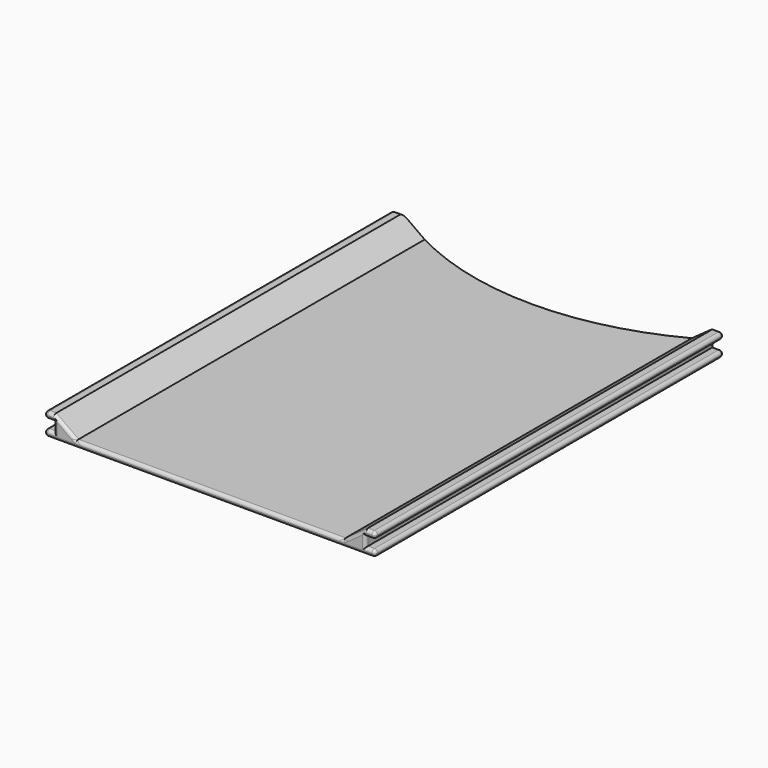
from build123d import *

# Parameters (mm, degrees)
F1_DEPTH       = 2
F2_W           = 10
F2_H           = 137
F3_DEPTH       = 5
F4_W           = 137
F4_H           = 3
F5_DEPTH       = 3
F6_W           = 137
F6_H           = 3
F7_DEPTH       = 3
F8_T4_DEPTH    = 173.1483869651
F8_T9_DEPTH    = 173.1483869651
F10_T1_DEPTH   = 134.9980686292
F10_T3_DEPTH   = 101.9980686292
F10_T5_DEPTH   = 1.9990343146
F10_T7_DEPTH   = 3
F10_T9_DEPTH   = 4.5014487279
F10_T11_DEPTH  = 4.5014487279
F10_T13_DEPTH  = 1.9990343146
F10_T15_DEPTH  = 11.5014487279
F10_T17_DEPTH  = 11.5014487279
F10_S21_W      = 1.1015022539
F10_S21_H      = 1.1015022539
F10_T22_DEPTH  = 1.101502254
F10_S27_W      = 1.1015022539
F10_S27_H      = 1.1015022539
F10_T28_DEPTH  = 1.101502254
F10_S33_W      = 1.1015022539
F10_S33_H      = 1.1015022539
F10_T34_DEPTH  = 1.101502254
F10_S39_W      = 1.1015022539
F10_S39_H      = 1.1015022539
F10_T40_DEPTH  = 1.101502254
F10_S45_W      = 1.1015022539
F10_S45_H      = 1.1015022539
F10_T46_DEPTH  = 1.101502254
F10_S51_W      = 1.1015022539
F10_S51_H      = 1.1015022539
F10_T52_DEPTH  = 1.101502254
F10_S57_W      = 1.1015022539
F10_S57_H      = 1.1015022539
F10_T58_DEPTH  = 1.101502254
F10_S63_W      = 1.1015022539
F10_S63_H      = 1.1015022539
F10_T64_DEPTH  = 1.101502254
F10_S69_W      = 1.1015022539
F10_S69_H      = 1.1015022539
F10_T70_DEPTH  = 1.101502254
F10_S75_W      = 1.1015022539
F10_S75_H      = 1.1015022539
F10_T76_DEPTH  = 1.101502254
F10_S81_W      = 1.1015022539
F10_S81_H      = 1.1015022539
F10_T82_DEPTH  = 1.101502254
F10_S87_W      = 1.1015022539
F10_S87_H      = 1.1015022539
F10_T88_DEPTH  = 1.101502254
F10_S93_W      = 1.1015022539
F10_S93_H      = 1.1015022539
F10_T94_DEPTH  = 1.101502254
F10_S99_W      = 1.1015022539
F10_S99_H      = 1.1015022539
F10_T100_DEPTH = 1.101502254
F10_S105_W     = 1.1015022539
F10_S105_H     = 1.1015022539
F10_T106_DEPTH = 1.101502254
F10_S111_W     = 1.1015022539
F10_S111_H     = 1.1015022539
F10_T112_DEPTH = 1.101502254
F10_T118_DEPTH = 13.6071540938
F10_T123_DEPTH = 89.0048288267
F10_T129_DEPTH = 13.6071540938
F10_T132_ANGLE = 58.8229405879
F10_T137_DEPTH = 4.5014487279
F10_T141_DEPTH = 5.5024144134
F10_T149_DEPTH = 5.5024144134
F10_T155_DEPTH = 4.5014487279
F10_T163_DEPTH = 13.6071540938
F10_T168_DEPTH = 89.0048288267
F10_T175_DEPTH = 13.6071540938
F10_T180_DEPTH = 89.0048288267
F10_T187_DEPTH = 5.5024144134
F10_T193_DEPTH = 4.5014487279
F10_T201_DEPTH = 4.5014487279
F10_T205_DEPTH = 5.5024144134
F10_T213_DEPTH = 4.5014487279
F10_T218_DEPTH = 5.5024144134
F10_T227_DEPTH = 5.5024144134
F10_T232_DEPTH = 4.5014487279
F10_T239_DEPTH = 4.5014487279
F10_T243_DEPTH = 5.5024144134
F10_T251_DEPTH = 5.5024144134
F10_T257_DEPTH = 4.5014487279


# Not quite as in the source:
# - a fillet or chamfer that OpenCascade refuses, or shapes differently, is made with other operations: its cross-section is extruded or revolved along the edge and cut away or added
# - two fillets or chamfers of one size are made in one step


with BuildPart() as f1:
    # F0 (on Top) → F1 (new body)
    with BuildSketch(Plane.XY):
        with BuildLine():
            Line((-52, -68.5), (0, -68.5))
            Line((0, -68.5), (52, -68.5))
            Line((52, -68.5), (52, 68.5))
            Line((52, 68.5), (42, 68.5))
            ThreePointArc((42, 68.5), (0, 58.0989949685), (-42, 68.5))
            Line((-42, 68.5), (-52, 68.5))
            Line((-52, 68.5), (-52, -68.5))
        make_face()
    extrude(amount=F1_DEPTH)

    # F2 (on face) → F3 (join)
    with BuildSketch(Plane.XY.offset(2)):
        with Locations((-47, 0)):
            Rectangle(F2_W, F2_H)
        with Locations((47, 0)):
            Rectangle(F2_W, F2_H)
    extrude(amount=F3_DEPTH)

    # F4 (on face) → F5 (cut)
    with BuildSketch(Plane(origin=(-52, 0, 0), x_dir=(0, -1, 0), z_dir=(-1, 0, 0))):
        with Locations((0, 3.5)):
            Rectangle(F4_W, F4_H)
    extrude(amount=-F5_DEPTH, mode=Mode.SUBTRACT)

    # F6 (on face) → F7 (cut)
    with BuildSketch(Plane.YZ.offset(52)):
        with Locations((0, 3.5)):
            Rectangle(F6_W, F6_H)
    extrude(amount=-F7_DEPTH, mode=Mode.SUBTRACT)

    # F8: chamfer of 7 x 5 on 2 edges, made by hand


with BuildPart() as f8_tool2:
    # F8_s3 → F8_t4 (new body)
    with BuildSketch(Plane.XZ.offset(86.5741934825)):
        Polygon((-49, 7), (-42, 2), (-42, 7), align=None)
    extrude(amount=-F8_T4_DEPTH)

    split(bisect_by=Plane.XY.offset(2), keep=Keep.TOP)


with BuildPart() as f1_1:
    add(f1.part)

    # F8_t1: cut F8_tool2
    add(f8_tool2.part, mode=Mode.SUBTRACT)


with BuildPart() as f8_tool7:
    # F8_s8 → F8_t9 (new body)
    with BuildSketch(Plane.XZ.offset(-86.5741934825)):
        Polygon((49, 7), (42, 2), (42, 7), align=None)
    extrude(amount=F8_T9_DEPTH)

    split(bisect_by=Plane.XY.offset(2), keep=Keep.TOP)


with BuildPart() as f1_2:
    add(f1_1.part)

    # F8_t6: cut F8_tool7
    add(f8_tool7.part, mode=Mode.SUBTRACT)

    # F10: fillet of radius 1 on 39 edges, made by hand

    # F10_s2 → F10_t1 (cut)
    with BuildSketch(Plane.XZ.offset(-67.4990343146)):
        with BuildLine():
            ThreePointArc((52.0004, 0.9990343146), (51.7071067812, 1.7071067812), (50.9990343146, 2.0004))
            Line((50.9990343146, 2.0004), (50.9990343146, 2.1005365685))
            ThreePointArc((50.9990343146, 2.1005365685), (51.4995171573, 2.1001365685), (52, 2.1001365685))
            Line((52, 2.1001365685), (52.1001365685, 2))
            ThreePointArc((52.1001365685, 2), (52.1001365685, 1.4995171573), (52.1005365685, 0.9990343146))
            Line((52.1005365685, 0.9990343146), (52.0004, 0.9990343146))
        make_face()
        with BuildLine():
            ThreePointArc((50.9990343146, -0.0004), (51.7071067812, 0.2928932188), (52.0004, 1.0009656854))
            Line((52.0004, 1.0009656854), (52.1005365685, 1.0009656854))
            ThreePointArc((52.1005365685, 1.0009656854), (52.1001365685, 0.5004828427), (52.1001365685, 0))
            Line((52.1001365685, 0), (52, -0.1001365685))
            ThreePointArc((52, -0.1001365685), (51.4995171573, -0.1001365685), (50.9990343146, -0.1005365685))
            Line((50.9990343146, -0.1005365685), (50.9990343146, -0.0004))
        make_face()
        with BuildLine():
            ThreePointArc((52.0004, 5.9990343146), (51.7071067812, 6.7071067812), (50.9990343146, 7.0004))
            Line((50.9990343146, 7.0004), (50.9990343146, 7.1005365685))
            ThreePointArc((50.9990343146, 7.1005365685), (51.4995171573, 7.1001365685), (52, 7.1001365685))
            Line((52, 7.1001365685), (52.1001365685, 7))
            ThreePointArc((52.1001365685, 7), (52.1001365685, 6.4995171573), (52.1005365685, 5.9990343146))
            Line((52.1005365685, 5.9990343146), (52.0004, 5.9990343146))
        make_face()
        with BuildLine():
            ThreePointArc((50.9990343146, 4.9996), (51.7071067812, 5.2928932188), (52.0004, 6.0009656854))
            Line((52.0004, 6.0009656854), (52.1005365685, 6.0009656854))
            ThreePointArc((52.1005365685, 6.0009656854), (52.1001365685, 5.5004828427), (52.1001365685, 5))
            Line((52.1001365685, 5), (52, 4.8998634315))
            ThreePointArc((52, 4.8998634315), (51.4995171573, 4.8998634315), (50.9990343146, 4.8994634315))
            Line((50.9990343146, 4.8994634315), (50.9990343146, 4.9996))
        make_face()
        with BuildLine():
            ThreePointArc((-52.0004, 5.9990343146), (-51.7071067812, 6.7071067812), (-50.9990343146, 7.0004))
            Line((-50.9990343146, 7.0004), (-50.9990343146, 7.1005365685))
            ThreePointArc((-50.9990343146, 7.1005365685), (-51.4995171573, 7.1001365685), (-52, 7.1001365685))
            Line((-52, 7.1001365685), (-52.1001365685, 7))
            ThreePointArc((-52.1001365685, 7), (-52.1001365685, 6.4995171573), (-52.1005365685, 5.9990343146))
            Line((-52.1005365685, 5.9990343146), (-52.0004, 5.9990343146))
        make_face()
        with BuildLine():
            ThreePointArc((-50.9990343146, 4.9996), (-51.7071067812, 5.2928932188), (-52.0004, 6.0009656854))
            Line((-52.0004, 6.0009656854), (-52.1005365685, 6.0009656854))
            ThreePointArc((-52.1005365685, 6.0009656854), (-52.1001365685, 5.5004828427), (-52.1001365685, 5))
            Line((-52.1001365685, 5), (-52, 4.8998634315))
            ThreePointArc((-52, 4.8998634315), (-51.4995171573, 4.8998634315), (-50.9990343146, 4.8994634315))
            Line((-50.9990343146, 4.8994634315), (-50.9990343146, 4.9996))
        make_face()
        with BuildLine():
            ThreePointArc((-52.0004, 0.9990343146), (-51.7071067812, 1.7071067812), (-50.9990343146, 2.0004))
            Line((-50.9990343146, 2.0004), (-50.9990343146, 2.1005365685))
            ThreePointArc((-50.9990343146, 2.1005365685), (-51.4995171573, 2.1001365685), (-52, 2.1001365685))
            Line((-52, 2.1001365685), (-52.1001365685, 2))
            ThreePointArc((-52.1001365685, 2), (-52.1001365685, 1.4995171573), (-52.1005365685, 0.9990343146))
            Line((-52.1005365685, 0.9990343146), (-52.0004, 0.9990343146))
        make_face()
        with BuildLine():
            ThreePointArc((-50.9990343146, -0.0004), (-51.7071067812, 0.2928932188), (-52.0004, 1.0009656854))
            Line((-52.0004, 1.0009656854), (-52.1005365685, 1.0009656854))
            ThreePointArc((-52.1005365685, 1.0009656854), (-52.1001365685, 0.5004828427), (-52.1001365685, 0))
            Line((-52.1001365685, 0), (-52, -0.1001365685))
            ThreePointArc((-52, -0.1001365685), (-51.4995171573, -0.1001365685), (-50.9990343146, -0.1005365685))
            Line((-50.9990343146, -0.1005365685), (-50.9990343146, -0.0004))
        make_face()
    extrude(amount=F10_T1_DEPTH, mode=Mode.SUBTRACT)

    # F10_s4 → F10_t3 (cut)
    with BuildSketch(Plane.YZ.offset(-50.9990343146)):
        with BuildLine():
            ThreePointArc((-67.4990343146, -0.0004), (-68.2071067812, 0.2928932188), (-68.5004, 1.0009656854))
            Line((-68.5004, 1.0009656854), (-68.6005365685, 1.0009656854))
            ThreePointArc((-68.6005365685, 1.0009656854), (-68.6001365685, 0.5004828427), (-68.6001365685, 0))
            Line((-68.6001365685, 0), (-68.5, -0.1001365685))
            ThreePointArc((-68.5, -0.1001365685), (-67.9995171573, -0.1001365685), (-67.4990343146, -0.1005365685))
            Line((-67.4990343146, -0.1005365685), (-67.4990343146, -0.0004))
        make_face()
    extrude(amount=F10_T3_DEPTH, mode=Mode.SUBTRACT)

    # F10_s6 → F10_t5 (cut)
    with BuildSketch(Plane.YZ.offset(49)):
        with BuildLine():
            ThreePointArc((-68.5004, 0.9990343146), (-68.2071067812, 1.7071067812), (-67.4990343146, 2.0004))
            Line((-67.4990343146, 2.0004), (-67.4990343146, 2.1005365685))
            ThreePointArc((-67.4990343146, 2.1005365685), (-67.9995171573, 2.1001365685), (-68.5, 2.1001365685))
            Line((-68.5, 2.1001365685), (-68.6001365685, 2))
            ThreePointArc((-68.6001365685, 2), (-68.6001365685, 1.4995171573), (-68.6005365685, 0.9990343146))
            Line((-68.6005365685, 0.9990343146), (-68.5004, 0.9990343146))
        make_face()
        with BuildLine():
            ThreePointArc((-68.5004, 6.0009656854), (-68.2071067812, 5.2928932188), (-67.4990343146, 4.9996))
            Line((-67.4990343146, 4.9996), (-67.4990343146, 4.8994634315))
            ThreePointArc((-67.4990343146, 4.8994634315), (-67.9995171573, 4.8998634315), (-68.5, 4.8998634315))
            Line((-68.5, 4.8998634315), (-68.6001365685, 5))
            ThreePointArc((-68.6001365685, 5), (-68.6001365685, 5.5004828427), (-68.6005365685, 6.0009656854))
            Line((-68.6005365685, 6.0009656854), (-68.5004, 6.0009656854))
        make_face()
        with BuildLine():
            ThreePointArc((68.5004, 6.0009656854), (68.2071067812, 5.2928932188), (67.4990343146, 4.9996))
            Line((67.4990343146, 4.9996), (67.4990343146, 4.8994634315))
            ThreePointArc((67.4990343146, 4.8994634315), (67.9995171573, 4.8998634315), (68.5, 4.8998634315))
            Line((68.5, 4.8998634315), (68.6001365685, 5))
            ThreePointArc((68.6001365685, 5), (68.6001365685, 5.5004828427), (68.6005365685, 6.0009656854))
            Line((68.6005365685, 6.0009656854), (68.5004, 6.0009656854))
        make_face()
        with BuildLine():
            ThreePointArc((68.5004, 0.9990343146), (68.2071067812, 1.7071067812), (67.4990343146, 2.0004))
            Line((67.4990343146, 2.0004), (67.4990343146, 2.1005365685))
            ThreePointArc((67.4990343146, 2.1005365685), (67.9995171573, 2.1001365685), (68.5, 2.1001365685))
            Line((68.5, 2.1001365685), (68.6001365685, 2))
            ThreePointArc((68.6001365685, 2), (68.6001365685, 1.4995171573), (68.6005365685, 0.9990343146))
            Line((68.6005365685, 0.9990343146), (68.5004, 0.9990343146))
        make_face()
    extrude(amount=F10_T5_DEPTH, mode=Mode.SUBTRACT)

    # F10_s8 → F10_t7 (cut)
    with BuildSketch(Plane.XY.offset(2)):
        with BuildLine():
            ThreePointArc((47.9990343146, -68.5004), (48.7071067812, -68.2071067812), (49.0004, -67.4990343146))
            Line((49.0004, -67.4990343146), (49.1005365685, -67.4990343146))
            ThreePointArc((49.1005365685, -67.4990343146), (49.1001365685, -67.9995171573), (49.1001365685, -68.5))
            Line((49.1001365685, -68.5), (49, -68.6001365685))
            ThreePointArc((49, -68.6001365685), (48.4995171573, -68.6001365685), (47.9990343146, -68.6005365685))
            Line((47.9990343146, -68.6005365685), (47.9990343146, -68.5004))
        make_face()
        with BuildLine():
            ThreePointArc((-49.0004, -67.4990343146), (-48.7071067812, -68.2071067812), (-47.9990343146, -68.5004))
            Line((-47.9990343146, -68.5004), (-47.9990343146, -68.6005365685))
            ThreePointArc((-47.9990343146, -68.6005365685), (-48.4995171573, -68.6001365685), (-49, -68.6001365685))
            Line((-49, -68.6001365685), (-49.1001365685, -68.5))
            ThreePointArc((-49.1001365685, -68.5), (-49.1001365685, -67.9995171573), (-49.1005365685, -67.4990343146))
            Line((-49.1005365685, -67.4990343146), (-49.0004, -67.4990343146))
        make_face()
        with BuildLine():
            ThreePointArc((47.9990343146, 68.5004), (48.7071067812, 68.2071067812), (49.0004, 67.4990343146))
            Line((49.0004, 67.4990343146), (49.1005365685, 67.4990343146))
            ThreePointArc((49.1005365685, 67.4990343146), (49.1001365685, 67.9995171573), (49.1001365685, 68.5))
            Line((49.1001365685, 68.5), (49, 68.6001365685))
            ThreePointArc((49, 68.6001365685), (48.4995171573, 68.6001365685), (47.9990343146, 68.6005365685))
            Line((47.9990343146, 68.6005365685), (47.9990343146, 68.5004))
        make_face()
        with BuildLine():
            ThreePointArc((-47.9990343146, 68.5004), (-48.7071067812, 68.2071067812), (-49.0004, 67.4990343146))
            Line((-49.0004, 67.4990343146), (-49.1005365685, 67.4990343146))
            ThreePointArc((-49.1005365685, 67.4990343146), (-49.1001365685, 67.9995171573), (-49.1001365685, 68.5))
            Line((-49.1001365685, 68.5), (-49, 68.6001365685))
            ThreePointArc((-49, 68.6001365685), (-48.4995171573, 68.6001365685), (-47.9990343146, 68.6005365685))
            Line((-47.9990343146, 68.6005365685), (-47.9990343146, 68.5004))
        make_face()
    extrude(amount=F10_T7_DEPTH, mode=Mode.SUBTRACT)

    # F10_s10 → F10_t9 (cut)
    with BuildSketch(Plane.YZ.offset(46.4975855866)):
        with BuildLine():
            ThreePointArc((-68.5004, 5.9990343146), (-68.2071067812, 6.7071067812), (-67.4990343146, 7.0004))
            Line((-67.4990343146, 7.0004), (-67.4990343146, 7.1005365685))
            ThreePointArc((-67.4990343146, 7.1005365685), (-67.9995171573, 7.1001365685), (-68.5, 7.1001365685))
            Line((-68.5, 7.1001365685), (-68.6001365685, 7))
            ThreePointArc((-68.6001365685, 7), (-68.6001365685, 6.4995171573), (-68.6005365685, 5.9990343146))
            Line((-68.6005365685, 5.9990343146), (-68.5004, 5.9990343146))
        make_face()
        with BuildLine():
            ThreePointArc((68.5004, 5.9990343146), (68.2071067812, 6.7071067812), (67.4990343146, 7.0004))
            Line((67.4990343146, 7.0004), (67.4990343146, 7.1005365685))
            ThreePointArc((67.4990343146, 7.1005365685), (67.9995171573, 7.1001365685), (68.5, 7.1001365685))
            Line((68.5, 7.1001365685), (68.6001365685, 7))
            ThreePointArc((68.6001365685, 7), (68.6001365685, 6.4995171573), (68.6005365685, 5.9990343146))
            Line((68.6005365685, 5.9990343146), (68.5004, 5.9990343146))
        make_face()
    extrude(amount=F10_T9_DEPTH, mode=Mode.SUBTRACT)

    # F10_s12 → F10_t11 (cut)
    with BuildSketch(Plane.YZ.offset(-50.9990343146)):
        with BuildLine():
            ThreePointArc((-67.4990343146, 7.0004), (-68.2071067812, 6.7071067812), (-68.5004, 5.9990343146))
            Line((-68.5004, 5.9990343146), (-68.6005365685, 5.9990343146))
            ThreePointArc((-68.6005365685, 5.9990343146), (-68.6001365685, 6.4995171573), (-68.6001365685, 7))
            Line((-68.6001365685, 7), (-68.5, 7.1001365685))
            ThreePointArc((-68.5, 7.1001365685), (-67.9995171573, 7.1001365685), (-67.4990343146, 7.1005365685))
            Line((-67.4990343146, 7.1005365685), (-67.4990343146, 7.0004))
        make_face()
        with BuildLine():
            ThreePointArc((68.5004, 5.9990343146), (68.2071067812, 6.7071067812), (67.4990343146, 7.0004))
            Line((67.4990343146, 7.0004), (67.4990343146, 7.1005365685))
            ThreePointArc((67.4990343146, 7.1005365685), (67.9995171573, 7.1001365685), (68.5, 7.1001365685))
            Line((68.5, 7.1001365685), (68.6001365685, 7))
            ThreePointArc((68.6001365685, 7), (68.6001365685, 6.4995171573), (68.6005365685, 5.9990343146))
            Line((68.6005365685, 5.9990343146), (68.5004, 5.9990343146))
        make_face()
    extrude(amount=F10_T11_DEPTH, mode=Mode.SUBTRACT)

    # F10_s14 → F10_t13 (cut)
    with BuildSketch(Plane.YZ.offset(-50.9990343146)):
        with BuildLine():
            ThreePointArc((-67.4990343146, 4.9996), (-68.2071067812, 5.2928932188), (-68.5004, 6.0009656854))
            Line((-68.5004, 6.0009656854), (-68.6005365685, 6.0009656854))
            ThreePointArc((-68.6005365685, 6.0009656854), (-68.6001365685, 5.5004828427), (-68.6001365685, 5))
            Line((-68.6001365685, 5), (-68.5, 4.8998634315))
            ThreePointArc((-68.5, 4.8998634315), (-67.9995171573, 4.8998634315), (-67.4990343146, 4.8994634315))
            Line((-67.4990343146, 4.8994634315), (-67.4990343146, 4.9996))
        make_face()
        with BuildLine():
            ThreePointArc((-67.4990343146, 2.0004), (-68.2071067812, 1.7071067812), (-68.5004, 0.9990343146))
            Line((-68.5004, 0.9990343146), (-68.6005365685, 0.9990343146))
            ThreePointArc((-68.6005365685, 0.9990343146), (-68.6001365685, 1.4995171573), (-68.6001365685, 2))
            Line((-68.6001365685, 2), (-68.5, 2.1001365685))
            ThreePointArc((-68.5, 2.1001365685), (-67.9995171573, 2.1001365685), (-67.4990343146, 2.1005365685))
            Line((-67.4990343146, 2.1005365685), (-67.4990343146, 2.0004))
        make_face()
        with BuildLine():
            ThreePointArc((68.5004, 0.9990343146), (68.2071067812, 1.7071067812), (67.4990343146, 2.0004))
            Line((67.4990343146, 2.0004), (67.4990343146, 2.1005365685))
            ThreePointArc((67.4990343146, 2.1005365685), (67.9995171573, 2.1001365685), (68.5, 2.1001365685))
            Line((68.5, 2.1001365685), (68.6001365685, 2))
            ThreePointArc((68.6001365685, 2), (68.6001365685, 1.4995171573), (68.6005365685, 0.9990343146))
            Line((68.6005365685, 0.9990343146), (68.5004, 0.9990343146))
        make_face()
        with BuildLine():
            ThreePointArc((68.5004, 6.0009656854), (68.2071067812, 5.2928932188), (67.4990343146, 4.9996))
            Line((67.4990343146, 4.9996), (67.4990343146, 4.8994634315))
            ThreePointArc((67.4990343146, 4.8994634315), (67.9995171573, 4.8998634315), (68.5, 4.8998634315))
            Line((68.5, 4.8998634315), (68.6001365685, 5))
            ThreePointArc((68.6001365685, 5), (68.6001365685, 5.5004828427), (68.6005365685, 6.0009656854))
            Line((68.6005365685, 6.0009656854), (68.5004, 6.0009656854))
        make_face()
    extrude(amount=F10_T13_DEPTH, mode=Mode.SUBTRACT)

    # F10_s16 → F10_t15 (cut)
    with BuildSketch(Plane.YZ.offset(39.4975855866)):
        with BuildLine():
            ThreePointArc((67.4990343146, -0.0004), (68.2071067812, 0.2928932188), (68.5004, 1.0009656854))
            Line((68.5004, 1.0009656854), (68.6005365685, 1.0009656854))
            ThreePointArc((68.6005365685, 1.0009656854), (68.6001365685, 0.5004828427), (68.6001365685, 0))
            Line((68.6001365685, 0), (68.5, -0.1001365685))
            ThreePointArc((68.5, -0.1001365685), (67.9995171573, -0.1001365685), (67.4990343146, -0.1005365685))
            Line((67.4990343146, -0.1005365685), (67.4990343146, -0.0004))
        make_face()
    extrude(amount=F10_T15_DEPTH, mode=Mode.SUBTRACT)

    # F10_s18 → F10_t17 (cut)
    with BuildSketch(Plane.YZ.offset(-50.9990343146)):
        with BuildLine():
            ThreePointArc((68.5004, 1.0009656854), (68.2071067812, 0.2928932188), (67.4990343146, -0.0004))
            Line((67.4990343146, -0.0004), (67.4990343146, -0.1005365685))
            ThreePointArc((67.4990343146, -0.1005365685), (67.9995171573, -0.1001365685), (68.5, -0.1001365685))
            Line((68.5, -0.1001365685), (68.6001365685, 0))
            ThreePointArc((68.6001365685, 0), (68.6001365685, 0.5004828427), (68.6005365685, 1.0009656854))
            Line((68.6005365685, 1.0009656854), (68.5004, 1.0009656854))
        make_face()
    extrude(amount=F10_T17_DEPTH, mode=Mode.SUBTRACT)


with BuildPart() as f10_tool20:
    # F10_s21 → F10_t22 (new body)
    with BuildSketch(Plane.XZ.offset(67.4990343146)):
        with Locations((51.5497854416, 1.5497854416)):
            Rectangle(F10_S21_W, F10_S21_H)
    extrude(amount=F10_T22_DEPTH)

    # F10_s23 → F10_t24 (revolve, cut)
    with BuildSketch(Plane(origin=(50.9990343146, -67.4990343146, 0.9990343146), x_dir=(-0.7071067812, 0, -0.7071067812), z_dir=(-0.7071067812, 0, 0.7071067812))):
        with BuildLine():
            ThreePointArc((0, -1.0013656854), (1.0013656854, 0), (0, 1.0013656854))
            Line((0, 1.0013656854), (0, -1.0013656854))
        make_face()
    revolve(axis=Axis((50.9990343146, -67.4990343146, 0.9990343146), (0, -1, 0)), mode=Mode.SUBTRACT)


with BuildPart() as f1_3:
    add(f1_2.part)

    # F10_t19: cut F10_tool20
    add(f10_tool20.part, mode=Mode.SUBTRACT)


with BuildPart() as f10_tool26:
    # F10_s27 → F10_t28 (new body)
    with BuildSketch(Plane.YZ.offset(50.9990343146)):
        with Locations((68.0497854416, 1.5497854416)):
            Rectangle(F10_S27_W, F10_S27_H)
    extrude(amount=F10_T28_DEPTH)

    # F10_s29 → F10_t30 (revolve, cut)
    with BuildSketch(Plane(origin=(50.9990343146, 67.4990343146, 0.9990343146), x_dir=(0, -0.7071067812, -0.7071067812), z_dir=(0, -0.7071067812, 0.7071067812))):
        with BuildLine():
            ThreePointArc((0, -1.0013656854), (1.0013656854, 0), (0, 1.0013656854))
            Line((0, 1.0013656854), (0, -1.0013656854))
        make_face()
    revolve(axis=Axis((50.9990343146, 67.4990343146, 0.9990343146), (1, 0, 0)), mode=Mode.SUBTRACT)


with BuildPart() as f1_4:
    add(f1_3.part)

    # F10_t25: cut F10_tool26
    add(f10_tool26.part, mode=Mode.SUBTRACT)


with BuildPart() as f10_tool32:
    # F10_s33 → F10_t34 (new body)
    with BuildSketch(Plane.XY.offset(1.0009656854)):
        with Locations((51.5497854416, -68.0497854416)):
            Rectangle(F10_S33_W, F10_S33_H)
    extrude(amount=-F10_T34_DEPTH)

    # F10_s35 → F10_t36 (revolve, cut)
    with BuildSketch(Plane(origin=(50.9990343146, -67.4990343146, 1.0009656854), x_dir=(-0.7071067812, 0.7071067812, 0), z_dir=(-0.7071067812, -0.7071067812, 0))):
        with BuildLine():
            ThreePointArc((0, -1.0013656854), (1.0013656854, 0), (0, 1.0013656854))
            Line((0, 1.0013656854), (0, -1.0013656854))
        make_face()
    revolve(axis=Axis((50.9990343146, -67.4990343146, 1.0009656854), (0, 0, -1)), mode=Mode.SUBTRACT)


with BuildPart() as f1_5:
    add(f1_4.part)

    # F10_t31: cut F10_tool32
    add(f10_tool32.part, mode=Mode.SUBTRACT)


with BuildPart() as f10_tool38:
    # F10_s39 → F10_t40 (new body)
    with BuildSketch(Plane.XY.offset(1.0009656854)):
        with Locations((51.5497854416, 68.0497854416)):
            Rectangle(F10_S39_W, F10_S39_H)
    extrude(amount=-F10_T40_DEPTH)

    # F10_s41 → F10_t42 (revolve, cut)
    with BuildSketch(Plane(origin=(50.9990343146, 67.4990343146, 1.0009656854), x_dir=(-0.7071067812, -0.7071067812, 0), z_dir=(0.7071067812, -0.7071067812, 0))):
        with BuildLine():
            ThreePointArc((0, -1.0013656854), (1.0013656854, 0), (0, 1.0013656854))
            Line((0, 1.0013656854), (0, -1.0013656854))
        make_face()
    revolve(axis=Axis((50.9990343146, 67.4990343146, 1.0009656854), (0, 0, -1)), mode=Mode.SUBTRACT)


with BuildPart() as f1_6:
    add(f1_5.part)

    # F10_t37: cut F10_tool38
    add(f10_tool38.part, mode=Mode.SUBTRACT)


with BuildPart() as f10_tool44:
    # F10_s45 → F10_t46 (new body)
    with BuildSketch(Plane.YZ.offset(50.9990343146)):
        with Locations((-68.0497854416, 6.5497854416)):
            Rectangle(F10_S45_W, F10_S45_H)
    extrude(amount=F10_T46_DEPTH)

    # F10_s47 → F10_t48 (revolve, cut)
    with BuildSketch(Plane(origin=(50.9990343146, -67.4990343146, 5.9990343146), x_dir=(0, 0.7071067812, -0.7071067812), z_dir=(0, -0.7071067812, -0.7071067812))):
        with BuildLine():
            ThreePointArc((0, -1.0013656854), (1.0013656854, 0), (0, 1.0013656854))
            Line((0, 1.0013656854), (0, -1.0013656854))
        make_face()
    revolve(axis=Axis((50.9990343146, -67.4990343146, 5.9990343146), (1, 0, 0)), mode=Mode.SUBTRACT)


with BuildPart() as f1_7:
    add(f1_6.part)

    # F10_t43: cut F10_tool44
    add(f10_tool44.part, mode=Mode.SUBTRACT)


with BuildPart() as f10_tool50:
    # F10_s51 → F10_t52 (new body)
    with BuildSketch(Plane.YZ.offset(50.9990343146)):
        with Locations((68.0497854416, 6.5497854416)):
            Rectangle(F10_S51_W, F10_S51_H)
    extrude(amount=F10_T52_DEPTH)

    # F10_s53 → F10_t54 (revolve, cut)
    with BuildSketch(Plane(origin=(50.9990343146, 67.4990343146, 5.9990343146), x_dir=(0, -0.7071067812, -0.7071067812), z_dir=(0, -0.7071067812, 0.7071067812))):
        with BuildLine():
            ThreePointArc((0, -1.0013656854), (1.0013656854, 0), (0, 1.0013656854))
            Line((0, 1.0013656854), (0, -1.0013656854))
        make_face()
    revolve(axis=Axis((50.9990343146, 67.4990343146, 5.9990343146), (1, 0, 0)), mode=Mode.SUBTRACT)


with BuildPart() as f1_8:
    add(f1_7.part)

    # F10_t49: cut F10_tool50
    add(f10_tool50.part, mode=Mode.SUBTRACT)


with BuildPart() as f10_tool56:
    # F10_s57 → F10_t58 (new body)
    with BuildSketch(Plane.XY.offset(6.0009656854)):
        with Locations((51.5497854416, 68.0497854416)):
            Rectangle(F10_S57_W, F10_S57_H)
    extrude(amount=-F10_T58_DEPTH)

    # F10_s59 → F10_t60 (revolve, cut)
    with BuildSketch(Plane(origin=(50.9990343146, 67.4990343146, 6.0009656854), x_dir=(-0.7071067812, -0.7071067812, 0), z_dir=(0.7071067812, -0.7071067812, 0))):
        with BuildLine():
            ThreePointArc((0, -1.0013656854), (1.0013656854, 0), (0, 1.0013656854))
            Line((0, 1.0013656854), (0, -1.0013656854))
        make_face()
    revolve(axis=Axis((50.9990343146, 67.4990343146, 6.0009656854), (0, 0, -1)), mode=Mode.SUBTRACT)


with BuildPart() as f1_9:
    add(f1_8.part)

    # F10_t55: cut F10_tool56
    add(f10_tool56.part, mode=Mode.SUBTRACT)


with BuildPart() as f10_tool62:
    # F10_s63 → F10_t64 (new body)
    with BuildSketch(Plane.XY.offset(6.0009656854)):
        with Locations((51.5497854416, -68.0497854416)):
            Rectangle(F10_S63_W, F10_S63_H)
    extrude(amount=-F10_T64_DEPTH)

    # F10_s65 → F10_t66 (revolve, cut)
    with BuildSketch(Plane(origin=(50.9990343146, -67.4990343146, 6.0009656854), x_dir=(-0.7071067812, 0.7071067812, 0), z_dir=(-0.7071067812, -0.7071067812, 0))):
        with BuildLine():
            ThreePointArc((0, -1.0013656854), (1.0013656854, 0), (0, 1.0013656854))
            Line((0, 1.0013656854), (0, -1.0013656854))
        make_face()
    revolve(axis=Axis((50.9990343146, -67.4990343146, 6.0009656854), (0, 0, -1)), mode=Mode.SUBTRACT)


with BuildPart() as f1_10:
    add(f1_9.part)

    # F10_t61: cut F10_tool62
    add(f10_tool62.part, mode=Mode.SUBTRACT)


with BuildPart() as f10_tool68:
    # F10_s69 → F10_t70 (new body)
    with BuildSketch(Plane.XZ.offset(-67.4990343146)):
        with Locations((-51.5497854416, 6.5497854416)):
            Rectangle(F10_S69_W, F10_S69_H)
    extrude(amount=-F10_T70_DEPTH)

    # F10_s71 → F10_t72 (revolve, cut)
    with BuildSketch(Plane(origin=(-50.9990343146, 67.4990343146, 5.9990343146), x_dir=(0.7071067812, 0, -0.7071067812), z_dir=(0.7071067812, 0, 0.7071067812))):
        with BuildLine():
            ThreePointArc((0, -1.0013656854), (1.0013656854, 0), (0, 1.0013656854))
            Line((0, 1.0013656854), (0, -1.0013656854))
        make_face()
    revolve(axis=Axis((-50.9990343146, 67.4990343146, 5.9990343146), (0, 1, 0)), mode=Mode.SUBTRACT)


with BuildPart() as f1_11:
    add(f1_10.part)

    # F10_t67: cut F10_tool68
    add(f10_tool68.part, mode=Mode.SUBTRACT)


with BuildPart() as f10_tool74:
    # F10_s75 → F10_t76 (new body)
    with BuildSketch(Plane.XZ.offset(67.4990343146)):
        with Locations((-51.5497854416, 6.5497854416)):
            Rectangle(F10_S75_W, F10_S75_H)
    extrude(amount=F10_T76_DEPTH)

    # F10_s77 → F10_t78 (revolve, cut)
    with BuildSketch(Plane(origin=(-50.9990343146, -67.4990343146, 5.9990343146), x_dir=(0.7071067812, 0, -0.7071067812), z_dir=(-0.7071067812, 0, -0.7071067812))):
        with BuildLine():
            ThreePointArc((0, -1.0013656854), (1.0013656854, 0), (0, 1.0013656854))
            Line((0, 1.0013656854), (0, -1.0013656854))
        make_face()
    revolve(axis=Axis((-50.9990343146, -67.4990343146, 5.9990343146), (0, -1, 0)), mode=Mode.SUBTRACT)


with BuildPart() as f1_12:
    add(f1_11.part)

    # F10_t73: cut F10_tool74
    add(f10_tool74.part, mode=Mode.SUBTRACT)


with BuildPart() as f10_tool80:
    # F10_s81 → F10_t82 (new body)
    with BuildSketch(Plane.XZ.offset(67.4990343146)):
        with Locations((-51.5497854416, 5.4502145584)):
            Rectangle(F10_S81_W, F10_S81_H)
    extrude(amount=F10_T82_DEPTH)

    # F10_s83 → F10_t84 (revolve, cut)
    with BuildSketch(Plane(origin=(-50.9990343146, -67.4990343146, 6.0009656854), x_dir=(0.7071067812, 0, 0.7071067812), z_dir=(0.7071067812, 0, -0.7071067812))):
        with BuildLine():
            ThreePointArc((0, -1.0013656854), (1.0013656854, 0), (0, 1.0013656854))
            Line((0, 1.0013656854), (0, -1.0013656854))
        make_face()
    revolve(axis=Axis((-50.9990343146, -67.4990343146, 6.0009656854), (0, -1, 0)), mode=Mode.SUBTRACT)


with BuildPart() as f1_13:
    add(f1_12.part)

    # F10_t79: cut F10_tool80
    add(f10_tool80.part, mode=Mode.SUBTRACT)


with BuildPart() as f10_tool86:
    # F10_s87 → F10_t88 (new body)
    with BuildSketch(Plane.XZ.offset(-67.4990343146)):
        with Locations((-51.5497854416, 5.4502145584)):
            Rectangle(F10_S87_W, F10_S87_H)
    extrude(amount=-F10_T88_DEPTH)

    # F10_s89 → F10_t90 (revolve, cut)
    with BuildSketch(Plane(origin=(-50.9990343146, 67.4990343146, 6.0009656854), x_dir=(0.7071067812, 0, 0.7071067812), z_dir=(-0.7071067812, 0, 0.7071067812))):
        with BuildLine():
            ThreePointArc((0, -1.0013656854), (1.0013656854, 0), (0, 1.0013656854))
            Line((0, 1.0013656854), (0, -1.0013656854))
        make_face()
    revolve(axis=Axis((-50.9990343146, 67.4990343146, 6.0009656854), (0, 1, 0)), mode=Mode.SUBTRACT)


with BuildPart() as f1_14:
    add(f1_13.part)

    # F10_t85: cut F10_tool86
    add(f10_tool86.part, mode=Mode.SUBTRACT)


with BuildPart() as f10_tool92:
    # F10_s93 → F10_t94 (new body)
    with BuildSketch(Plane.XZ.offset(-67.4990343146)):
        with Locations((-51.5497854416, 1.5497854416)):
            Rectangle(F10_S93_W, F10_S93_H)
    extrude(amount=-F10_T94_DEPTH)

    # F10_s95 → F10_t96 (revolve, cut)
    with BuildSketch(Plane(origin=(-50.9990343146, 67.4990343146, 0.9990343146), x_dir=(0.7071067812, 0, -0.7071067812), z_dir=(0.7071067812, 0, 0.7071067812))):
        with BuildLine():
            ThreePointArc((0, -1.0013656854), (1.0013656854, 0), (0, 1.0013656854))
            Line((0, 1.0013656854), (0, -1.0013656854))
        make_face()
    revolve(axis=Axis((-50.9990343146, 67.4990343146, 0.9990343146), (0, 1, 0)), mode=Mode.SUBTRACT)


with BuildPart() as f1_15:
    add(f1_14.part)

    # F10_t91: cut F10_tool92
    add(f10_tool92.part, mode=Mode.SUBTRACT)


with BuildPart() as f10_tool98:
    # F10_s99 → F10_t100 (new body)
    with BuildSketch(Plane.XZ.offset(67.4990343146)):
        with Locations((-51.5497854416, 1.5497854416)):
            Rectangle(F10_S99_W, F10_S99_H)
    extrude(amount=F10_T100_DEPTH)

    # F10_s101 → F10_t102 (revolve, cut)
    with BuildSketch(Plane(origin=(-50.9990343146, -67.4990343146, 0.9990343146), x_dir=(0.7071067812, 0, -0.7071067812), z_dir=(-0.7071067812, 0, -0.7071067812))):
        with BuildLine():
            ThreePointArc((0, -1.0013656854), (1.0013656854, 0), (0, 1.0013656854))
            Line((0, 1.0013656854), (0, -1.0013656854))
        make_face()
    revolve(axis=Axis((-50.9990343146, -67.4990343146, 0.9990343146), (0, -1, 0)), mode=Mode.SUBTRACT)


with BuildPart() as f1_16:
    add(f1_15.part)

    # F10_t97: cut F10_tool98
    add(f10_tool98.part, mode=Mode.SUBTRACT)


with BuildPart() as f10_tool104:
    # F10_s105 → F10_t106 (new body)
    with BuildSketch(Plane.XY.offset(1.0009656854)):
        with Locations((-51.5497854416, -68.0497854416)):
            Rectangle(F10_S105_W, F10_S105_H)
    extrude(amount=-F10_T106_DEPTH)

    # F10_s107 → F10_t108 (revolve, cut)
    with BuildSketch(Plane(origin=(-50.9990343146, -67.4990343146, 1.0009656854), x_dir=(0.7071067812, 0.7071067812, 0), z_dir=(-0.7071067812, 0.7071067812, 0))):
        with BuildLine():
            ThreePointArc((0, -1.0013656854), (1.0013656854, 0), (0, 1.0013656854))
            Line((0, 1.0013656854), (0, -1.0013656854))
        make_face()
    revolve(axis=Axis((-50.9990343146, -67.4990343146, 1.0009656854), (0, 0, -1)), mode=Mode.SUBTRACT)


with BuildPart() as f1_17:
    add(f1_16.part)

    # F10_t103: cut F10_tool104
    add(f10_tool104.part, mode=Mode.SUBTRACT)


with BuildPart() as f10_tool110:
    # F10_s111 → F10_t112 (new body)
    with BuildSketch(Plane.XZ.offset(-67.4990343146)):
        with Locations((-51.5497854416, 0.4502145584)):
            Rectangle(F10_S111_W, F10_S111_H)
    extrude(amount=-F10_T112_DEPTH)

    # F10_s113 → F10_t114 (revolve, cut)
    with BuildSketch(Plane(origin=(-50.9990343146, 67.4990343146, 1.0009656854), x_dir=(0.7071067812, 0, 0.7071067812), z_dir=(-0.7071067812, 0, 0.7071067812))):
        with BuildLine():
            ThreePointArc((0, -1.0013656854), (1.0013656854, 0), (0, 1.0013656854))
            Line((0, 1.0013656854), (0, -1.0013656854))
        make_face()
    revolve(axis=Axis((-50.9990343146, 67.4990343146, 1.0009656854), (0, 1, 0)), mode=Mode.SUBTRACT)


with BuildPart() as f1_18:
    add(f1_17.part)

    # F10_t109: cut F10_tool110
    add(f10_tool110.part, mode=Mode.SUBTRACT)


with BuildPart() as f10_tool116:
    # F10_s117 → F10_t118 (new body)
    with BuildSketch(Plane(origin=(37.7930551237, 0, 26.9950393741), x_dir=(0, 1, 0), z_dir=(-0.8137334712, 0, -0.5812381937))):
        with BuildLine():
            ThreePointArc((-68.5004, 23.7855028792), (-68.2071067812, 23.0774304126), (-67.4990343146, 22.7841371938))
            Line((-67.4990343146, 22.7841371938), (-67.4990343146, 22.6840006252))
            ThreePointArc((-67.4990343146, 22.6840006252), (-67.9995171573, 22.6844006252), (-68.5, 22.6844006252))
            Line((-68.5, 22.6844006252), (-68.6001365685, 22.7845371938))
            ThreePointArc((-68.6001365685, 22.7845371938), (-68.6001365685, 23.2850200365), (-68.6005365685, 23.7855028792))
            Line((-68.6005365685, 23.7855028792), (-68.5004, 23.7855028792))
        make_face()
    extrude(amount=F10_T118_DEPTH)

    split(bisect_by=Plane.XY.offset(2), keep=Keep.TOP)


with BuildPart() as f1_19:
    add(f1_18.part)

    # F10_t115: cut F10_tool116
    add(f10_tool116.part, mode=Mode.SUBTRACT)


with BuildPart() as f10_tool121:
    # F10_s122 → F10_t123 (new body)
    with BuildSketch(Plane.YZ.offset(44.5024144134)):
        with BuildLine():
            ThreePointArc((-68.5004, 0.9990343146), (-68.2071067812, 1.7071067812), (-67.4990343146, 2.0004))
            Line((-67.4990343146, 2.0004), (-67.4990343146, 2.1005365685))
            ThreePointArc((-67.4990343146, 2.1005365685), (-67.9995171573, 2.1001365685), (-68.5, 2.1001365685))
            Line((-68.5, 2.1001365685), (-68.6001365685, 2))
            ThreePointArc((-68.6001365685, 2), (-68.6001365685, 1.4995171573), (-68.6005365685, 0.9990343146))
            Line((-68.6005365685, 0.9990343146), (-68.5004, 0.9990343146))
        make_face()
    extrude(amount=-F10_T123_DEPTH)

    split(bisect_by=Plane(origin=(-13.2432432432, 0, -18.5405405405), x_dir=(0, 1, 0), z_dir=(0.5812381937, 0, 0.8137334712)), keep=Keep.TOP)

    split(bisect_by=Plane(origin=(13.2432432432, 0, -18.5405405405), x_dir=(0, 1, 0), z_dir=(-0.5812381937, 0, 0.8137334712)), keep=Keep.TOP)


with BuildPart() as f1_20:
    add(f1_19.part)

    # F10_t120: cut F10_tool121
    add(f10_tool121.part, mode=Mode.SUBTRACT)


with BuildPart() as f10_tool127:
    # F10_s128 → F10_t129 (new body)
    with BuildSketch(Plane(origin=(-26.7204583898, 0, 19.086041707), x_dir=(0, 1, 0), z_dir=(-0.8137334712, 0, 0.5812381937))):
        with BuildLine():
            ThreePointArc((-67.4990343146, 22.7841371938), (-68.2071067812, 23.0774304126), (-68.5004, 23.7855028792))
            Line((-68.5004, 23.7855028792), (-68.6005365685, 23.7855028792))
            ThreePointArc((-68.6005365685, 23.7855028792), (-68.6001365685, 23.2850200365), (-68.6001365685, 22.7845371938))
            Line((-68.6001365685, 22.7845371938), (-68.5, 22.6844006252))
            ThreePointArc((-68.5, 22.6844006252), (-67.9995171573, 22.6844006252), (-67.4990343146, 22.6840006252))
            Line((-67.4990343146, 22.6840006252), (-67.4990343146, 22.7841371938))
        make_face()
    extrude(amount=F10_T129_DEPTH)

    split(bisect_by=Plane.XY.offset(2), keep=Keep.TOP)


with BuildPart() as f1_21:
    add(f1_20.part)

    # F10_t126: cut F10_tool127
    add(f10_tool127.part, mode=Mode.SUBTRACT)

    # F10_s131 → F10_t132 (revolve, cut)
    with BuildSketch(Plane(origin=(63.3546473233, 35.7152211742, 0), x_dir=(0, 0, 1), z_dir=(0.8711155175, 0.4910781559, 0))):
        with BuildLine():
            ThreePointArc((-0.0004, -38.0103669552), (0.2928932188, -38.7184394218), (1.0009656854, -39.0117326406))
            Line((1.0009656854, -39.0117326406), (1.0009656854, -39.1118692092))
            ThreePointArc((1.0009656854, -39.1118692092), (0.5004828427, -39.1114692092), (0, -39.1114692092))
            Line((0, -39.1114692092), (-0.1001365685, -39.0113326406))
            ThreePointArc((-0.1001365685, -39.0113326406), (-0.1001365685, -38.5108497979), (-0.1005365685, -38.0103669552))
            Line((-0.1005365685, -38.0103669552), (-0.0004, -38.0103669552))
        make_face()
    revolve(axis=Axis((0, 148.0989949685, 0), (0, 0, -1)), revolution_arc=F10_T132_ANGLE, mode=Mode.SUBTRACT)


with BuildPart() as f10_tool135:
    # F10_s136 → F10_t137 (new body)
    with BuildSketch(Plane.YZ.offset(50.9990343146)):
        with BuildLine():
            ThreePointArc((-68.5004, 0.9990343146), (-68.2071067812, 1.7071067812), (-67.4990343146, 2.0004))
            Line((-67.4990343146, 2.0004), (-67.4990343146, 2.1005365685))
            ThreePointArc((-67.4990343146, 2.1005365685), (-67.9995171573, 2.1001365685), (-68.5, 2.1001365685))
            Line((-68.5, 2.1001365685), (-68.6001365685, 2))
            ThreePointArc((-68.6001365685, 2), (-68.6001365685, 1.4995171573), (-68.6005365685, 0.9990343146))
            Line((-68.6005365685, 0.9990343146), (-68.5004, 0.9990343146))
        make_face()
    extrude(amount=-F10_T137_DEPTH)

    split(bisect_by=Plane.YZ.offset(49), keep=Keep.BOTTOM)


with BuildPart() as f10_tool139:
    # F10_s140 → F10_t141 (new body)
    with BuildSketch(Plane.XY.offset(5)):
        with BuildLine():
            ThreePointArc((47.9990343146, -68.5004), (48.7071067812, -68.2071067812), (49.0004, -67.4990343146))
            Line((49.0004, -67.4990343146), (49.1005365685, -67.4990343146))
            ThreePointArc((49.1005365685, -67.4990343146), (49.1001365685, -67.9995171573), (49.1001365685, -68.5))
            Line((49.1001365685, -68.5), (49, -68.6001365685))
            ThreePointArc((49, -68.6001365685), (48.4995171573, -68.6001365685), (47.9990343146, -68.6005365685))
            Line((47.9990343146, -68.6005365685), (47.9990343146, -68.5004))
        make_face()
    extrude(amount=-F10_T141_DEPTH)

    split(bisect_by=Plane.XY, keep=Keep.TOP)

    split(bisect_by=Plane.XY.offset(2), keep=Keep.BOTTOM)


with BuildPart() as f10_tool135_1:
    add(f10_tool135.part)

    # F10_t144: intersect F10_tool139
    add(f10_tool139.part, mode=Mode.INTERSECT)


with BuildPart() as f1_22:
    add(f1_21.part)

    # F10_t133: cut F10_tool135
    add(f10_tool135_1.part, mode=Mode.SUBTRACT)


with BuildPart() as f10_tool147:
    # F10_s148 → F10_t149 (new body)
    with BuildSketch(Plane.XY.offset(7.5024144134)):
        with BuildLine():
            ThreePointArc((47.9990343146, -68.5004), (48.7071067812, -68.2071067812), (49.0004, -67.4990343146))
            Line((49.0004, -67.4990343146), (49.1005365685, -67.4990343146))
            ThreePointArc((49.1005365685, -67.4990343146), (49.1001365685, -67.9995171573), (49.1001365685, -68.5))
            Line((49.1001365685, -68.5), (49, -68.6001365685))
            ThreePointArc((49, -68.6001365685), (48.4995171573, -68.6001365685), (47.9990343146, -68.6005365685))
            Line((47.9990343146, -68.6005365685), (47.9990343146, -68.5004))
        make_face()
    extrude(amount=-F10_T149_DEPTH)

    split(bisect_by=Plane.XY.offset(5), keep=Keep.TOP)

    split(bisect_by=Plane.XY.offset(7), keep=Keep.BOTTOM)

    split(bisect_by=Plane(origin=(13.2432432432, 0, -18.5405405405), x_dir=(0, 1, 0), z_dir=(0.5812381937, 0, -0.8137334712)), keep=Keep.TOP)


with BuildPart() as f10_tool153:
    # F10_s154 → F10_t155 (new body)
    with BuildSketch(Plane.YZ.offset(50.9990343146)):
        with BuildLine():
            ThreePointArc((-68.5004, 6.0009656854), (-68.2071067812, 5.2928932188), (-67.4990343146, 4.9996))
            Line((-67.4990343146, 4.9996), (-67.4990343146, 4.8994634315))
            ThreePointArc((-67.4990343146, 4.8994634315), (-67.9995171573, 4.8998634315), (-68.5, 4.8998634315))
            Line((-68.5, 4.8998634315), (-68.6001365685, 5))
            ThreePointArc((-68.6001365685, 5), (-68.6001365685, 5.5004828427), (-68.6005365685, 6.0009656854))
            Line((-68.6005365685, 6.0009656854), (-68.5004, 6.0009656854))
        make_face()
    extrude(amount=-F10_T155_DEPTH)

    split(bisect_by=Plane.YZ.offset(49), keep=Keep.BOTTOM)

    split(bisect_by=Plane(origin=(13.2432432432, 0, -18.5405405405), x_dir=(0, 1, 0), z_dir=(0.5812381937, 0, -0.8137334712)), keep=Keep.TOP)


with BuildPart() as f10_tool147_1:
    add(f10_tool147.part)

    # F10_t158: intersect F10_tool153
    add(f10_tool153.part, mode=Mode.INTERSECT)


with BuildPart() as f1_23:
    add(f1_22.part)

    # F10_t145: cut F10_tool147
    add(f10_tool147_1.part, mode=Mode.SUBTRACT)


with BuildPart() as f10_tool161:
    # F10_s162 → F10_t163 (new body)
    with BuildSketch(Plane(origin=(37.7930551237, 0, 26.9950393741), x_dir=(0, 1, 0), z_dir=(-0.8137334712, 0, -0.5812381937))):
        with BuildLine():
            ThreePointArc((-68.5004, 23.7855028792), (-68.2071067812, 23.0774304126), (-67.4990343146, 22.7841371938))
            Line((-67.4990343146, 22.7841371938), (-67.4990343146, 22.6840006252))
            ThreePointArc((-67.4990343146, 22.6840006252), (-67.9995171573, 22.6844006252), (-68.5, 22.6844006252))
            Line((-68.5, 22.6844006252), (-68.6001365685, 22.7845371938))
            ThreePointArc((-68.6001365685, 22.7845371938), (-68.6001365685, 23.2850200365), (-68.6005365685, 23.7855028792))
            Line((-68.6005365685, 23.7855028792), (-68.5004, 23.7855028792))
        make_face()
    extrude(amount=F10_T163_DEPTH)

    split(bisect_by=Plane.XY, keep=Keep.TOP)

    split(bisect_by=Plane.XY.offset(2), keep=Keep.BOTTOM)


with BuildPart() as f10_tool166:
    # F10_s167 → F10_t168 (new body)
    with BuildSketch(Plane.YZ.offset(44.5024144134)):
        with BuildLine():
            ThreePointArc((-68.5004, 0.9990343146), (-68.2071067812, 1.7071067812), (-67.4990343146, 2.0004))
            Line((-67.4990343146, 2.0004), (-67.4990343146, 2.1005365685))
            ThreePointArc((-67.4990343146, 2.1005365685), (-67.9995171573, 2.1001365685), (-68.5, 2.1001365685))
            Line((-68.5, 2.1001365685), (-68.6001365685, 2))
            ThreePointArc((-68.6001365685, 2), (-68.6001365685, 1.4995171573), (-68.6005365685, 0.9990343146))
            Line((-68.6005365685, 0.9990343146), (-68.5004, 0.9990343146))
        make_face()
    extrude(amount=-F10_T168_DEPTH)

    split(bisect_by=Plane(origin=(13.2432432432, 0, -18.5405405405), x_dir=(0, 1, 0), z_dir=(0.5812381937, 0, -0.8137334712)), keep=Keep.TOP)


with BuildPart() as f10_tool161_1:
    add(f10_tool161.part)

    # F10_t170: intersect F10_tool166
    add(f10_tool166.part, mode=Mode.INTERSECT)


with BuildPart() as f1_24:
    add(f1_23.part)

    # F10_t159: cut F10_tool161
    add(f10_tool161_1.part, mode=Mode.SUBTRACT)


with BuildPart() as f10_tool173:
    # F10_s174 → F10_t175 (new body)
    with BuildSketch(Plane(origin=(-26.7204583898, 0, 19.086041707), x_dir=(0, 1, 0), z_dir=(-0.8137334712, 0, 0.5812381937))):
        with BuildLine():
            ThreePointArc((-67.4990343146, 22.7841371938), (-68.2071067812, 23.0774304126), (-68.5004, 23.7855028792))
            Line((-68.5004, 23.7855028792), (-68.6005365685, 23.7855028792))
            ThreePointArc((-68.6005365685, 23.7855028792), (-68.6001365685, 23.2850200365), (-68.6001365685, 22.7845371938))
            Line((-68.6001365685, 22.7845371938), (-68.5, 22.6844006252))
            ThreePointArc((-68.5, 22.6844006252), (-67.9995171573, 22.6844006252), (-67.4990343146, 22.6840006252))
            Line((-67.4990343146, 22.6840006252), (-67.4990343146, 22.7841371938))
        make_face()
    extrude(amount=F10_T175_DEPTH)

    split(bisect_by=Plane.XY, keep=Keep.TOP)

    split(bisect_by=Plane.XY.offset(2), keep=Keep.BOTTOM)


with BuildPart() as f10_tool178:
    # F10_s179 → F10_t180 (new body)
    with BuildSketch(Plane.YZ.offset(44.5024144134)):
        with BuildLine():
            ThreePointArc((-68.5004, 0.9990343146), (-68.2071067812, 1.7071067812), (-67.4990343146, 2.0004))
            Line((-67.4990343146, 2.0004), (-67.4990343146, 2.1005365685))
            ThreePointArc((-67.4990343146, 2.1005365685), (-67.9995171573, 2.1001365685), (-68.5, 2.1001365685))
            Line((-68.5, 2.1001365685), (-68.6001365685, 2))
            ThreePointArc((-68.6001365685, 2), (-68.6001365685, 1.4995171573), (-68.6005365685, 0.9990343146))
            Line((-68.6005365685, 0.9990343146), (-68.5004, 0.9990343146))
        make_face()
    extrude(amount=-F10_T180_DEPTH)

    split(bisect_by=Plane(origin=(-13.2432432432, 0, -18.5405405405), x_dir=(0, 1, 0), z_dir=(-0.5812381937, 0, -0.8137334712)), keep=Keep.TOP)


with BuildPart() as f10_tool173_1:
    add(f10_tool173.part)

    # F10_t182: intersect F10_tool178
    add(f10_tool178.part, mode=Mode.INTERSECT)


with BuildPart() as f1_25:
    add(f1_24.part)

    # F10_t171: cut F10_tool173
    add(f10_tool173_1.part, mode=Mode.SUBTRACT)


with BuildPart() as f10_tool185:
    # F10_s186 → F10_t187 (new body)
    with BuildSketch(Plane.XY.offset(2)):
        with BuildLine():
            ThreePointArc((-49.0004, -67.4990343146), (-48.7071067812, -68.2071067812), (-47.9990343146, -68.5004))
            Line((-47.9990343146, -68.5004), (-47.9990343146, -68.6005365685))
            ThreePointArc((-47.9990343146, -68.6005365685), (-48.4995171573, -68.6001365685), (-49, -68.6001365685))
            Line((-49, -68.6001365685), (-49.1001365685, -68.5))
            ThreePointArc((-49.1001365685, -68.5), (-49.1001365685, -67.9995171573), (-49.1005365685, -67.4990343146))
            Line((-49.1005365685, -67.4990343146), (-49.0004, -67.4990343146))
        make_face()
    extrude(amount=F10_T187_DEPTH)

    split(bisect_by=Plane.XY.offset(5), keep=Keep.TOP)

    split(bisect_by=Plane.XY.offset(7), keep=Keep.BOTTOM)

    split(bisect_by=Plane(origin=(-13.2432432432, 0, -18.5405405405), x_dir=(0, 1, 0), z_dir=(-0.5812381937, 0, -0.8137334712)), keep=Keep.TOP)


with BuildPart() as f10_tool191:
    # F10_s192 → F10_t193 (new body)
    with BuildSketch(Plane.YZ.offset(-50.9990343146)):
        with BuildLine():
            ThreePointArc((-67.4990343146, 4.9996), (-68.2071067812, 5.2928932188), (-68.5004, 6.0009656854))
            Line((-68.5004, 6.0009656854), (-68.6005365685, 6.0009656854))
            ThreePointArc((-68.6005365685, 6.0009656854), (-68.6001365685, 5.5004828427), (-68.6001365685, 5))
            Line((-68.6001365685, 5), (-68.5, 4.8998634315))
            ThreePointArc((-68.5, 4.8998634315), (-67.9995171573, 4.8998634315), (-67.4990343146, 4.8994634315))
            Line((-67.4990343146, 4.8994634315), (-67.4990343146, 4.9996))
        make_face()
    extrude(amount=F10_T193_DEPTH)

    split(bisect_by=Plane.YZ.offset(-49), keep=Keep.TOP)

    split(bisect_by=Plane(origin=(-13.2432432432, 0, -18.5405405405), x_dir=(0, 1, 0), z_dir=(-0.5812381937, 0, -0.8137334712)), keep=Keep.TOP)


with BuildPart() as f10_tool185_1:
    add(f10_tool185.part)

    # F10_t196: intersect F10_tool191
    add(f10_tool191.part, mode=Mode.INTERSECT)


with BuildPart() as f1_26:
    add(f1_25.part)

    # F10_t183: cut F10_tool185
    add(f10_tool185_1.part, mode=Mode.SUBTRACT)


with BuildPart() as f10_tool199:
    # F10_s200 → F10_t201 (new body)
    with BuildSketch(Plane.YZ.offset(-50.9990343146)):
        with BuildLine():
            ThreePointArc((-67.4990343146, 2.0004), (-68.2071067812, 1.7071067812), (-68.5004, 0.9990343146))
            Line((-68.5004, 0.9990343146), (-68.6005365685, 0.9990343146))
            ThreePointArc((-68.6005365685, 0.9990343146), (-68.6001365685, 1.4995171573), (-68.6001365685, 2))
            Line((-68.6001365685, 2), (-68.5, 2.1001365685))
            ThreePointArc((-68.5, 2.1001365685), (-67.9995171573, 2.1001365685), (-67.4990343146, 2.1005365685))
            Line((-67.4990343146, 2.1005365685), (-67.4990343146, 2.0004))
        make_face()
    extrude(amount=F10_T201_DEPTH)

    split(bisect_by=Plane.YZ.offset(-49), keep=Keep.TOP)


with BuildPart() as f10_tool203:
    # F10_s204 → F10_t205 (new body)
    with BuildSketch(Plane.XY.offset(-0.5024144134)):
        with BuildLine():
            ThreePointArc((-49.0004, -67.4990343146), (-48.7071067812, -68.2071067812), (-47.9990343146, -68.5004))
            Line((-47.9990343146, -68.5004), (-47.9990343146, -68.6005365685))
            ThreePointArc((-47.9990343146, -68.6005365685), (-48.4995171573, -68.6001365685), (-49, -68.6001365685))
            Line((-49, -68.6001365685), (-49.1001365685, -68.5))
            ThreePointArc((-49.1001365685, -68.5), (-49.1001365685, -67.9995171573), (-49.1005365685, -67.4990343146))
            Line((-49.1005365685, -67.4990343146), (-49.0004, -67.4990343146))
        make_face()
    extrude(amount=F10_T205_DEPTH)

    split(bisect_by=Plane.XY, keep=Keep.TOP)

    split(bisect_by=Plane.XY.offset(2), keep=Keep.BOTTOM)


with BuildPart() as f10_tool199_1:
    add(f10_tool199.part)

    # F10_t208: intersect F10_tool203
    add(f10_tool203.part, mode=Mode.INTERSECT)


with BuildPart() as f1_27:
    add(f1_26.part)

    # F10_t197: cut F10_tool199
    add(f10_tool199_1.part, mode=Mode.SUBTRACT)


with BuildPart() as f10_tool211:
    # F10_s212 → F10_t213 (new body)
    with BuildSketch(Plane.YZ.offset(50.9990343146)):
        with BuildLine():
            ThreePointArc((68.5004, 6.0009656854), (68.2071067812, 5.2928932188), (67.4990343146, 4.9996))
            Line((67.4990343146, 4.9996), (67.4990343146, 4.8994634315))
            ThreePointArc((67.4990343146, 4.8994634315), (67.9995171573, 4.8998634315), (68.5, 4.8998634315))
            Line((68.5, 4.8998634315), (68.6001365685, 5))
            ThreePointArc((68.6001365685, 5), (68.6001365685, 5.5004828427), (68.6005365685, 6.0009656854))
            Line((68.6005365685, 6.0009656854), (68.5004, 6.0009656854))
        make_face()
    extrude(amount=-F10_T213_DEPTH)

    split(bisect_by=Plane.YZ.offset(49), keep=Keep.BOTTOM)

    split(bisect_by=Plane(origin=(13.2432432432, 0, -18.5405405405), x_dir=(0, 1, 0), z_dir=(0.5812381937, 0, -0.8137334712)), keep=Keep.TOP)


with BuildPart() as f10_tool216:
    # F10_s217 → F10_t218 (new body)
    with BuildSketch(Plane.XY.offset(2)):
        with BuildLine():
            ThreePointArc((47.9990343146, 68.5004), (48.7071067812, 68.2071067812), (49.0004, 67.4990343146))
            Line((49.0004, 67.4990343146), (49.1005365685, 67.4990343146))
            ThreePointArc((49.1005365685, 67.4990343146), (49.1001365685, 67.9995171573), (49.1001365685, 68.5))
            Line((49.1001365685, 68.5), (49, 68.6001365685))
            ThreePointArc((49, 68.6001365685), (48.4995171573, 68.6001365685), (47.9990343146, 68.6005365685))
            Line((47.9990343146, 68.6005365685), (47.9990343146, 68.5004))
        make_face()
    extrude(amount=F10_T218_DEPTH)

    split(bisect_by=Plane.XY.offset(5), keep=Keep.TOP)

    split(bisect_by=Plane.XY.offset(7), keep=Keep.BOTTOM)

    split(bisect_by=Plane(origin=(13.2432432432, 0, -18.5405405405), x_dir=(0, 1, 0), z_dir=(0.5812381937, 0, -0.8137334712)), keep=Keep.TOP)


with BuildPart() as f10_tool211_1:
    add(f10_tool211.part)

    # F10_t222: intersect F10_tool216
    add(f10_tool216.part, mode=Mode.INTERSECT)


with BuildPart() as f1_28:
    add(f1_27.part)

    # F10_t209: cut F10_tool211
    add(f10_tool211_1.part, mode=Mode.SUBTRACT)


with BuildPart() as f10_tool225:
    # F10_s226 → F10_t227 (new body)
    with BuildSketch(Plane.XY.offset(-0.5024144134)):
        with BuildLine():
            ThreePointArc((47.9990343146, 68.5004), (48.7071067812, 68.2071067812), (49.0004, 67.4990343146))
            Line((49.0004, 67.4990343146), (49.1005365685, 67.4990343146))
            ThreePointArc((49.1005365685, 67.4990343146), (49.1001365685, 67.9995171573), (49.1001365685, 68.5))
            Line((49.1001365685, 68.5), (49, 68.6001365685))
            ThreePointArc((49, 68.6001365685), (48.4995171573, 68.6001365685), (47.9990343146, 68.6005365685))
            Line((47.9990343146, 68.6005365685), (47.9990343146, 68.5004))
        make_face()
    extrude(amount=F10_T227_DEPTH)

    split(bisect_by=Plane.XY, keep=Keep.TOP)

    split(bisect_by=Plane.XY.offset(2), keep=Keep.BOTTOM)


with BuildPart() as f10_tool230:
    # F10_s231 → F10_t232 (new body)
    with BuildSketch(Plane.YZ.offset(50.9990343146)):
        with BuildLine():
            ThreePointArc((68.5004, 0.9990343146), (68.2071067812, 1.7071067812), (67.4990343146, 2.0004))
            Line((67.4990343146, 2.0004), (67.4990343146, 2.1005365685))
            ThreePointArc((67.4990343146, 2.1005365685), (67.9995171573, 2.1001365685), (68.5, 2.1001365685))
            Line((68.5, 2.1001365685), (68.6001365685, 2))
            ThreePointArc((68.6001365685, 2), (68.6001365685, 1.4995171573), (68.6005365685, 0.9990343146))
            Line((68.6005365685, 0.9990343146), (68.5004, 0.9990343146))
        make_face()
    extrude(amount=-F10_T232_DEPTH)

    split(bisect_by=Plane.YZ.offset(49), keep=Keep.BOTTOM)


with BuildPart() as f10_tool225_1:
    add(f10_tool225.part)

    # F10_t234: intersect F10_tool230
    add(f10_tool230.part, mode=Mode.INTERSECT)


with BuildPart() as f1_29:
    add(f1_28.part)

    # F10_t223: cut F10_tool225
    add(f10_tool225_1.part, mode=Mode.SUBTRACT)


with BuildPart() as f10_tool237:
    # F10_s238 → F10_t239 (new body)
    with BuildSketch(Plane.YZ.offset(-50.9990343146)):
        with BuildLine():
            ThreePointArc((68.5004, 0.9990343146), (68.2071067812, 1.7071067812), (67.4990343146, 2.0004))
            Line((67.4990343146, 2.0004), (67.4990343146, 2.1005365685))
            ThreePointArc((67.4990343146, 2.1005365685), (67.9995171573, 2.1001365685), (68.5, 2.1001365685))
            Line((68.5, 2.1001365685), (68.6001365685, 2))
            ThreePointArc((68.6001365685, 2), (68.6001365685, 1.4995171573), (68.6005365685, 0.9990343146))
            Line((68.6005365685, 0.9990343146), (68.5004, 0.9990343146))
        make_face()
    extrude(amount=F10_T239_DEPTH)

    split(bisect_by=Plane.YZ.offset(-49), keep=Keep.TOP)


with BuildPart() as f10_tool241:
    # F10_s242 → F10_t243 (new body)
    with BuildSketch(Plane.XY.offset(5)):
        with BuildLine():
            ThreePointArc((-47.9990343146, 68.5004), (-48.7071067812, 68.2071067812), (-49.0004, 67.4990343146))
            Line((-49.0004, 67.4990343146), (-49.1005365685, 67.4990343146))
            ThreePointArc((-49.1005365685, 67.4990343146), (-49.1001365685, 67.9995171573), (-49.1001365685, 68.5))
            Line((-49.1001365685, 68.5), (-49, 68.6001365685))
            ThreePointArc((-49, 68.6001365685), (-48.4995171573, 68.6001365685), (-47.9990343146, 68.6005365685))
            Line((-47.9990343146, 68.6005365685), (-47.9990343146, 68.5004))
        make_face()
    extrude(amount=-F10_T243_DEPTH)

    split(bisect_by=Plane.XY, keep=Keep.TOP)

    split(bisect_by=Plane.XY.offset(2), keep=Keep.BOTTOM)


with BuildPart() as f10_tool237_1:
    add(f10_tool237.part)

    # F10_t246: intersect F10_tool241
    add(f10_tool241.part, mode=Mode.INTERSECT)


with BuildPart() as f1_30:
    add(f1_29.part)

    # F10_t235: cut F10_tool237
    add(f10_tool237_1.part, mode=Mode.SUBTRACT)


with BuildPart() as f10_tool249:
    # F10_s250 → F10_t251 (new body)
    with BuildSketch(Plane.XY.offset(7.5024144134)):
        with BuildLine():
            ThreePointArc((-47.9990343146, 68.5004), (-48.7071067812, 68.2071067812), (-49.0004, 67.4990343146))
            Line((-49.0004, 67.4990343146), (-49.1005365685, 67.4990343146))
            ThreePointArc((-49.1005365685, 67.4990343146), (-49.1001365685, 67.9995171573), (-49.1001365685, 68.5))
            Line((-49.1001365685, 68.5), (-49, 68.6001365685))
            ThreePointArc((-49, 68.6001365685), (-48.4995171573, 68.6001365685), (-47.9990343146, 68.6005365685))
            Line((-47.9990343146, 68.6005365685), (-47.9990343146, 68.5004))
        make_face()
    extrude(amount=-F10_T251_DEPTH)

    split(bisect_by=Plane.XY.offset(5), keep=Keep.TOP)

    split(bisect_by=Plane.XY.offset(7), keep=Keep.BOTTOM)

    split(bisect_by=Plane(origin=(-13.2432432432, 0, -18.5405405405), x_dir=(0, 1, 0), z_dir=(-0.5812381937, 0, -0.8137334712)), keep=Keep.TOP)


with BuildPart() as f10_tool255:
    # F10_s256 → F10_t257 (new body)
    with BuildSketch(Plane.YZ.offset(-50.9990343146)):
        with BuildLine():
            ThreePointArc((68.5004, 6.0009656854), (68.2071067812, 5.2928932188), (67.4990343146, 4.9996))
            Line((67.4990343146, 4.9996), (67.4990343146, 4.8994634315))
            ThreePointArc((67.4990343146, 4.8994634315), (67.9995171573, 4.8998634315), (68.5, 4.8998634315))
            Line((68.5, 4.8998634315), (68.6001365685, 5))
            ThreePointArc((68.6001365685, 5), (68.6001365685, 5.5004828427), (68.6005365685, 6.0009656854))
            Line((68.6005365685, 6.0009656854), (68.5004, 6.0009656854))
        make_face()
    extrude(amount=F10_T257_DEPTH)

    split(bisect_by=Plane.YZ.offset(-49), keep=Keep.TOP)

    split(bisect_by=Plane(origin=(-13.2432432432, 0, -18.5405405405), x_dir=(0, 1, 0), z_dir=(-0.5812381937, 0, -0.8137334712)), keep=Keep.TOP)


with BuildPart() as f10_tool249_1:
    add(f10_tool249.part)

    # F10_t260: intersect F10_tool255
    add(f10_tool255.part, mode=Mode.INTERSECT)


with BuildPart() as f1_31:
    add(f1_30.part)

    # F10_t247: cut F10_tool249
    add(f10_tool249_1.part, mode=Mode.SUBTRACT)


solid = f1_31.part
